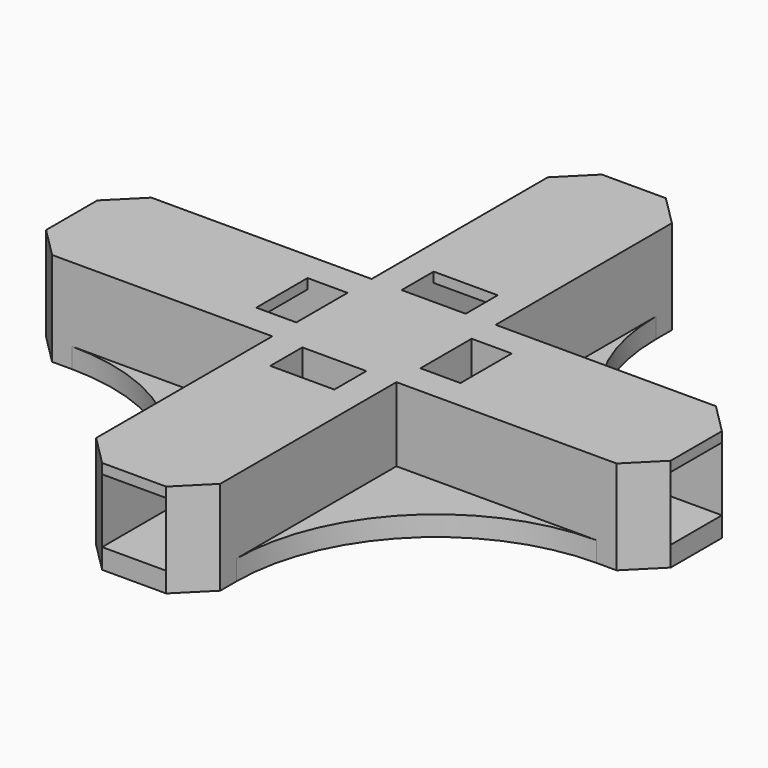
from build123d import *

# Parameters (mm, degrees)
F0_W     = 1.6
F0_H     = 12.5
F0_W_2   = 12.5
F0_H_2   = 1.6
F1_DEPTH = 1
F2_R     = 10
F3_DEPTH = 3.2
F4_COUNT = 4
F5_W     = 3.2
F5_H     = 2
F6_DEPTH = 0.5
F7_COUNT = 4


# Not quite as in the source:
# - a feature names something its author has since deleted; it is built from what else it names


with BuildPart() as f1:
    # F0 (on Top) → F1 (new body)
    with BuildSketch(Plane.XY):
        Polygon((3.1, 14.1), (1.6, 15.6), (1.6, 3.1), (1.6, 1.6), (3.1, 1.6), (15.6, 1.6), (14.1, 3.1), (3.1, 3.1), align=None)
        with Locations((0.8, 9.35)):
            Rectangle(F0_W, F0_H)
        Polygon((1.6, 1.6), (1.6, 3.1), (0, 3.1), (0, 0), (3.1, 0), (3.1, 1.6), align=None)
        with Locations((9.35, 0.8)):
            Rectangle(F0_W_2, F0_H_2)
    extrude(amount=-F1_DEPTH)

    # F2
    f2_edges = [f1.edges().sort_by_distance(p)[0] for p in [
        (3.1, 3.1, -0.5),
    ]]
    fillet(f2_edges, radius=F2_R)

    # F0 (on Top) → F3 (join)
    with BuildSketch(Plane.XY):
        Polygon((3.1, 14.1), (1.6, 15.6), (1.6, 3.1), (1.6, 1.6), (3.1, 1.6), (15.6, 1.6), (14.1, 3.1), (3.1, 3.1), align=None)
        Polygon((1.6, 1.6), (1.6, 3.1), (0, 3.1), (0, 0), (3.1, 0), (3.1, 1.6), align=None)
    extrude(amount=F3_DEPTH)

    # F4: F1 ×4 about axis
    f4_axis = Axis((0, 0, -0.5), (0, 0, 1))


with BuildPart() as f1_1:
    add(f1.part)
    for i in range(1, F4_COUNT):
        add(f1.part.rotate(f4_axis, i * 360 / F4_COUNT))



with BuildPart() as f6:
    # F5 (on face) → F6 (new body)
    with BuildSketch(Plane.XY.offset(3.2)):
        Polygon((1.6, 15.6), (-1.6, 15.6), (-3.1, 14.1), (-3.1, 3.1), (0, 0), (3.1, 3.1), (3.1, 14.1), align=None)
        with Locations((0, 4.1)):
            Rectangle(F5_W, F5_H, mode=Mode.SUBTRACT)
    extrude(amount=F6_DEPTH)


with BuildPart() as f1_2:
    add(f1_1.part)

    add(f6.part)  # F7 merges F6
    # F7: F6 ×4 about axis
    f7_axis = Axis((0, 0, 3.45), (0, 0, -1))
    for i in range(1, F7_COUNT):
        add(f6.part.rotate(f7_axis, i * 360 / F7_COUNT))


solid = f1_2.part
